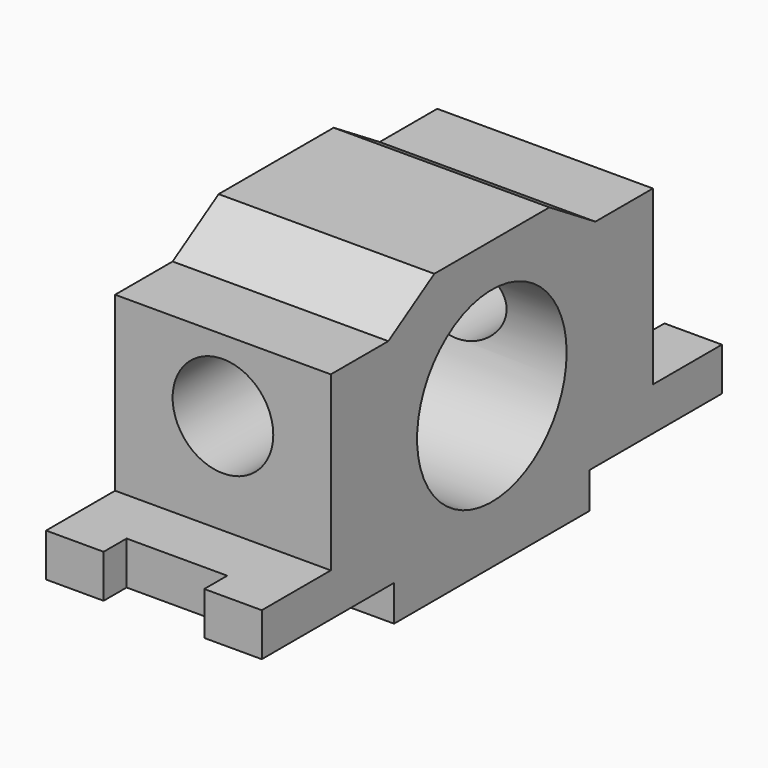
from build123d import *

# Parameters (mm, degrees)
F1_DEPTH = 15
F2_R     = 13
F3_DEPTH = 30.001
F4_W     = 14
F4_H     = 4
F5_DEPTH = 11.001
F6_R     = 7
F7_DEPTH = 68.001


# Not quite as in the source:
# - a pattern or mirror of a feature is missing from the dataset's text; its kind, count and spacing are read off the source's solid


with BuildPart() as f1:
    # F0 (on Right) → F1 (new body, symmetric)
    with BuildSketch(Plane.YZ):
        Polygon((-17, 0), (0, 0), (17, 0), (17, 5), (40, 5), (40, 11), (28, 11), (28, 35), (18, 35), (10, 40), (0, 40), (-10, 40), (-18, 35), (-28, 35), (-28, 11), (-40, 11), (-40, 5), (-17, 5), align=None)
    extrude(amount=F1_DEPTH, both=True)

    # F2 (on face) → F3 (cut, through all)
    with BuildSketch(Plane.YZ.offset(15)):
        with Locations((0, 21)):
            Circle(F2_R)
    extrude(amount=-F3_DEPTH, mode=Mode.SUBTRACT)

    # F4 (on face) → F5 (cut, through all)
    with BuildSketch(Plane.XY.offset(11)):
        with Locations((0, -38)):
            Rectangle(F4_W, F4_H)
    f5 = extrude(amount=-F5_DEPTH, mode=Mode.SUBTRACT)

    # F5_copies: F5 across plane
    add(f5.mirror(Plane.ZX), mode=Mode.SUBTRACT)

    # F6 (on face) → F7 (cut, through all)
    with BuildSketch(Plane.XZ.offset(28)):
        with Locations((0, 25)):
            Circle(F6_R)
    extrude(amount=-F7_DEPTH, mode=Mode.SUBTRACT)


solid = f1.part
